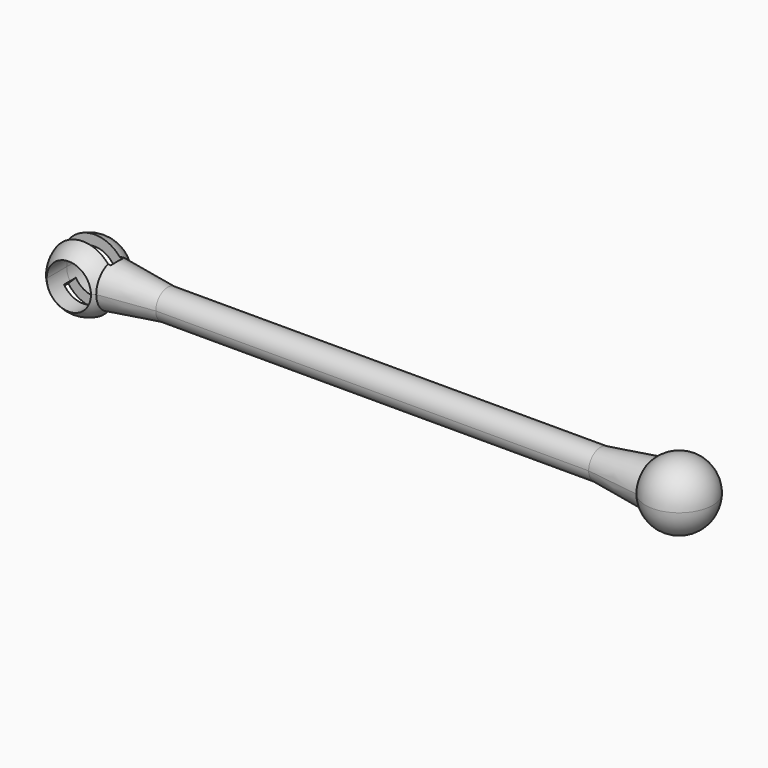
from build123d import *
from build123d import SkipClean  # not in build123d's __all__

# Parameters (mm, degrees)
F2_W           = 30
F2_H           = 1.5
F3_ANGLE_BACK  = 90
F3_ANGLE       = 180
F5_ANGLE_BACK  = 90
F5_ANGLE       = 180
F7_ANGLE_BACK  = 90
F7_ANGLE       = 180
F9_R           = 2.25
F10_DEPTH      = 3.401
F10_DEPTH_BACK = 3.401
F12_DEPTH      = 0.75


with BuildPart() as f3:
    # F2 (on Front) → F3 (revolve)
    with BuildSketch(Plane.XZ, mode=Mode.PRIVATE) as f3_sk:
        with Locations((-15, 0.75)):
            Rectangle(F2_W, F2_H)
    revolve(f3_sk.sketch.rotate(Axis((0, 0, 0), (1, 0, 0)), -F3_ANGLE_BACK), axis=Axis((0, 0, 0), (1, 0, 0)), revolution_arc=F3_ANGLE)

    # F4 (on Front) → F5 (revolve)
    with BuildSketch(Plane.XZ, mode=Mode.PRIVATE) as f5_sk:
        with BuildLine():
            Line((-33.4, 0), (-26.6, 0))
            ThreePointArc((-26.6, 0), (-30, 3.4), (-33.4, 0))
        make_face()
    revolve(f5_sk.sketch.rotate(Axis((0, 0, 0), (1, 0, 0)), -F5_ANGLE_BACK), axis=Axis((0, 0, 0), (1, 0, 0)), revolution_arc=F5_ANGLE)

    # F6 (on Front) → F7 (revolve)
    with BuildSketch(Plane.XZ, mode=Mode.PRIVATE) as f7_sk:
        Polygon((-27.4509805807, 2.25), (-30, 2.25), (-30, 0), (-22, 0), (-22, 1.5), align=None)
    revolve(f7_sk.sketch.rotate(Axis((0, 0, 0), (1, 0, 0)), -F7_ANGLE_BACK), axis=Axis((0, 0, 0), (1, 0, 0)), revolution_arc=F7_ANGLE)

    # F8: F3 across plane


with BuildPart() as f3_1:
    add(f3.part, clean=False)
    add(f3.part.mirror(Plane.YZ), clean=False)

    # F9 (on Front) → F10 (cut, two sides)
    with BuildSketch(Plane.XZ) as f10_sk:
        with Locations((-30, 0)):
            Circle(F9_R)
    extrude(amount=-F10_DEPTH, mode=Mode.SUBTRACT)
    extrude(f10_sk.sketch, amount=F10_DEPTH_BACK, mode=Mode.SUBTRACT)

    # F11 (on Front) → F12 (cut, symmetric)
    with BuildSketch(Plane.XZ):
        Polygon((-34.15, 3.4), (-30.75, 0), (-29.25, 0), (-25.85, 3.4), align=None)
    extrude(amount=F12_DEPTH, both=True, mode=Mode.SUBTRACT)

    # F13: F3 across plane


with BuildPart() as f3_2:
    add(f3_1.part, clean=False)
    with SkipClean():  # cleaning this boolean's faces spoils the solid; the shape is the same uncleaned
        add(f3_1.part.mirror(Plane.XY), clean=False)


solid = f3_2.part
